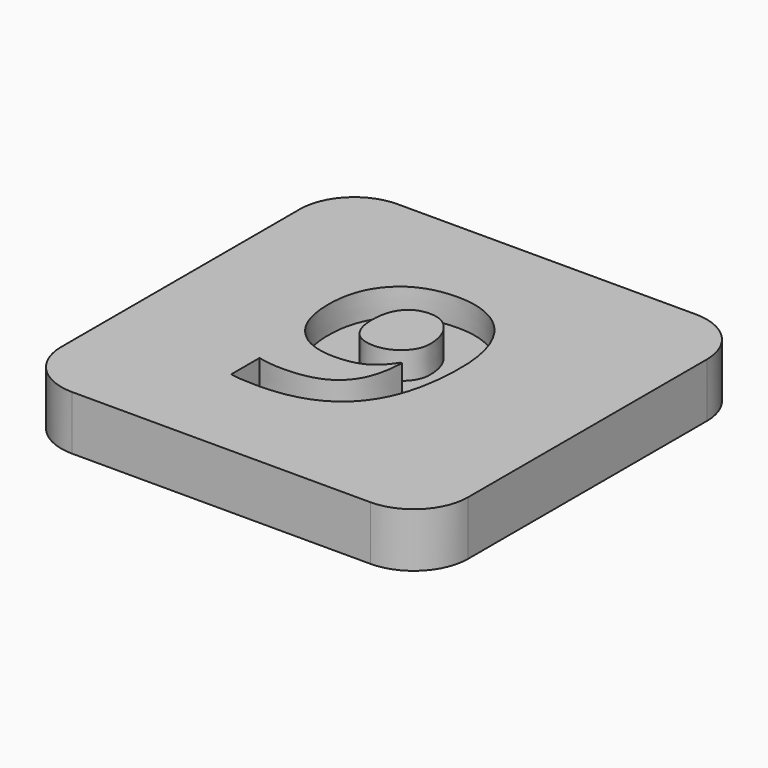
from build123d import *

# Parameters (mm, degrees)
F0_W         = 38.1
F0_H         = 38.1
F1_DEPTH     = 5.08
F2_TEXT_SIZE = 27.4737389496
F3_DEPTH     = 2.54
F4_R         = 5.08


# Not quite as in the source:
# - Text() gives the source's letters only with a copy of the font that has no kerning and outlines rounded to 1/6400 em; it was checked with that copy


with BuildPart() as f1:
    # F0 (on Top) → F1 (new body)
    with BuildSketch(Plane.XY):
        Rectangle(F0_W, F0_H)
    extrude(amount=F1_DEPTH)

    # F2 (on face) → F3 (cut)
    with BuildSketch(Plane.XY.offset(5.08)):
        with Locations((-8.89, -9.525)):
            Text('9', F2_TEXT_SIZE, font='Open Sans', font_style=FontStyle.BOLD, text_align=(TextAlign.LEFT, TextAlign.BOTTOM))
    extrude(amount=-F3_DEPTH, mode=Mode.SUBTRACT)

    # F4
    f4_edges = [f1.edges().sort_by_distance(p)[0] for p in [
        (-19.05, -19.05, 2.54),
        (19.05, -19.05, 2.54),
        (19.05, 19.05, 2.54),
        (-19.05, 19.05, 2.54),
    ]]
    fillet(f4_edges, radius=F4_R)


solid = f1.part
